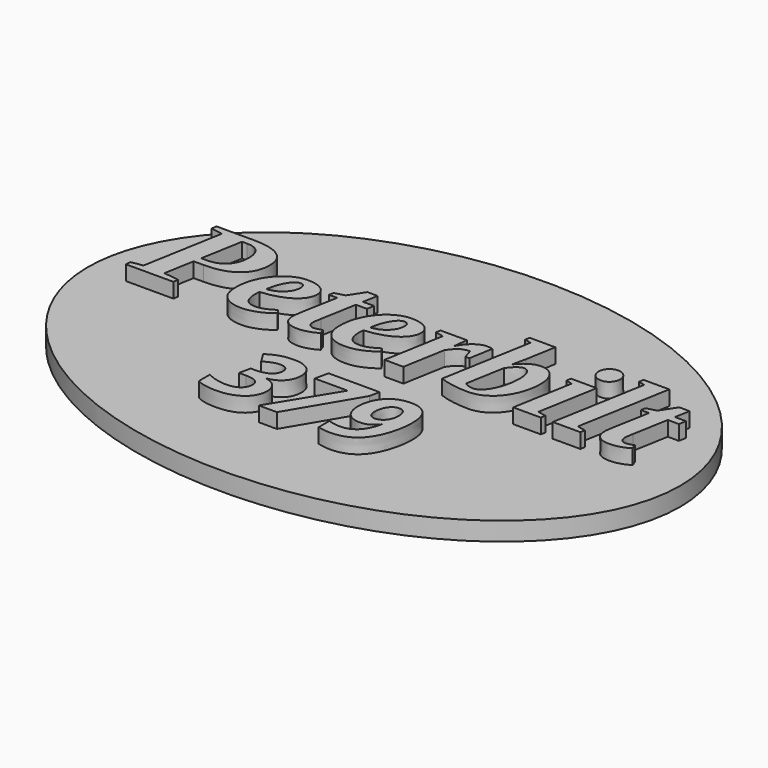
from build123d import *

# Parameters (mm, degrees)
F1_DEPTH       = 3.175
F2_TEXT_SIZE   = 24.6944444444
F2_TEXT_SIZE_2 = 18.3875898882
F3_DEPTH       = 2.54


# Not quite as in the source:
# - Text() gives the source's letters only with a copy of the font that has no kerning and outlines rounded to 1/6400 em; it was checked with that copy


with BuildPart() as f1:
    # F0 (on Top) → F1 (new body)
    with BuildSketch(Plane.XY):
        with BuildLine():
            add(Edge.make_bspline(
                [(50.8, 0), (50.8, 60.4918744543), (-25.4, 30.2459372272), (-101.6, 0), (-25.4, -30.2459372272), (50.8, -60.4918744543), (50.8, 0)],
                knots=[0, 0, 0, 2.0943951024, 2.0943951024, 4.1887902048, 4.1887902048, 6.2831853072, 6.2831853072, 6.2831853072], degree=2, weights=[1, 0.5, 1, 0.5, 1, 0.5, 1]))
        make_face()
    extrude(amount=F1_DEPTH)

    # F2 (on face) → F3 (join)
    with BuildSketch(Plane.XY.offset(3.175)):
        with Locations((-44.2898719618, 0)):
            Text('Peterbilt', F2_TEXT_SIZE, font='Tinos', font_style=FontStyle.BOLDITALIC, text_align=(TextAlign.LEFT, TextAlign.BOTTOM))
        with Locations((-15.6265783441, -20.8590647195)):
            Text('379', F2_TEXT_SIZE_2, font='Open Sans', font_style=FontStyle.BOLDITALIC, text_align=(TextAlign.LEFT, TextAlign.BOTTOM))
    extrude(amount=F3_DEPTH)


solid = f1.part
